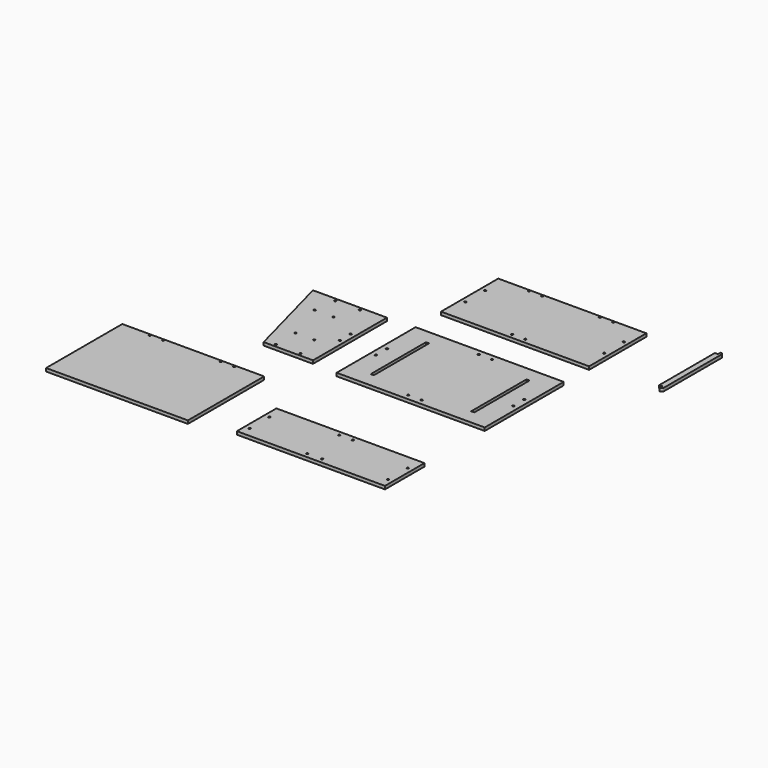
from build123d import *

# Parameters (mm, degrees)
F1_R     = 2
F4_DEPTH = 6.35
F0_R     = 2
F3_R     = 2
F2_R     = 2
F5_DEPTH = 6.35
F6_R     = 2
F7_DEPTH = 6.35


# Not quite as in the source:
# - a feature names something its author has since deleted; it is built from what else it names


with BuildPart() as f4:
    # F1 (on Top) → F4 (new body)
    with BuildSketch(Plane.XY):
        Polygon((1.8228454292, -180.5016371835), (-119.6771545708, -180.5016371835), (-119.6771545708, -210.5016371835), (-119.6771545708, -260.5016371835), (-119.6771545708, -280.5016371835), (30.3228454292, -280.5016371835), (180.3228454292, -280.5016371835), (180.3228454292, -180.5016371835), (58.8228454292, -180.5016371835), (28.8228454292, -180.5016371835), (15.3228454292, -180.5016371835), align=None)
        with Locations((-109.8271545708, -260.5016371835)):
            Circle(F1_R, mode=Mode.SUBTRACT)
        with Locations((15.3228454292, -271.0016371835)):
            Circle(F1_R, mode=Mode.SUBTRACT)
        with Locations((45.0311610582, -270.556012449)):
            Circle(F1_R, mode=Mode.SUBTRACT)
        with Locations((170.4728454292, -260.5016371835)):
            Circle(F1_R, mode=Mode.SUBTRACT)
        with Locations((-109.8271545708, -210.5016371835)):
            Circle(F1_R, mode=Mode.SUBTRACT)
        with Locations((15.3228454292, -190.0016371835)):
            Circle(F1_R, mode=Mode.SUBTRACT)
        with Locations((170.4728454292, -210.5016371835)):
            Circle(F1_R, mode=Mode.SUBTRACT)
        with Locations((42.6017076852, -189.5924542496)):
            Circle(F1_R, mode=Mode.SUBTRACT)
    extrude(amount=F4_DEPTH)


with BuildPart() as f4b:
    # F0 (on Top) → F4, piece 2 (new body)
    with BuildSketch(Plane.XY):
        Polygon((28.5, 174.3550467463), (-121.5, 174.3550467463), (-121.5, 88.3550467463), (-121.5, 60.3550467463), (-121.5, -25.6449532537), (0, -25.6449532537), (57, -25.6449532537), (178.5, -25.6449532537), (178.5, 174.3550467463), align=None)
        with Locations((-110.65, 60.3550467463)):
            Circle(F0_R, mode=Mode.SUBTRACT)
        Polygon((-76.5, 144.3550467463), (-70.15, 144.3550467463), (-70.15, 4.3550467463), (-76.5, 4.3550467463), (-76.5, 44.3550467463), (-76.5, 74.3550467463), align=None, mode=Mode.SUBTRACT)
        with Locations((15, -14.7949532537)):
            Circle(F0_R, mode=Mode.SUBTRACT)
        with Locations((42, -14.7949532537)):
            Circle(F0_R, mode=Mode.SUBTRACT)
        with Locations((-110.65, 88.3550467463)):
            Circle(F0_R, mode=Mode.SUBTRACT)
        with BuildLine():
            ThreePointArc((17, 163.5050467463), (13.5857864376, 162.0908331839), (15, 165.5050467463))
            ThreePointArc((15, 165.5050467463), (16.4142135624, 164.9192603087), (17, 163.5050467463))
        make_face(mode=Mode.SUBTRACT)
        with Locations((42, 163.5050467463)):
            Circle(F0_R, mode=Mode.SUBTRACT)
        Polygon((127.15, 4.3550467463), (127.15, 144.3550467463), (133.5, 144.3550467463), (133.5, 74.3550467463), (133.5, 44.3550467463), (133.5, 4.3550467463), align=None, mode=Mode.SUBTRACT)
        with Locations((167.65, 60.3550467463)):
            Circle(F0_R, mode=Mode.SUBTRACT)
        with Locations((167.65, 88.3550467463)):
            Circle(F0_R, mode=Mode.SUBTRACT)
    extrude(amount=F4_DEPTH)

    # F0 (on Top) → F5 (join)
    with BuildSketch(Plane.XY):
        Polygon((28.5, 174.3550467463), (-121.5, 174.3550467463), (-121.5, 88.3550467463), (-121.5, 60.3550467463), (-121.5, -25.6449532537), (0, -25.6449532537), (57, -25.6449532537), (178.5, -25.6449532537), (178.5, 174.3550467463), align=None)
        with Locations((-110.65, 60.3550467463)):
            Circle(F0_R, mode=Mode.SUBTRACT)
        Polygon((-76.5, 144.3550467463), (-70.15, 144.3550467463), (-70.15, 4.3550467463), (-76.5, 4.3550467463), (-76.5, 44.3550467463), (-76.5, 74.3550467463), align=None, mode=Mode.SUBTRACT)
        with Locations((15, -14.7949532537)):
            Circle(F0_R, mode=Mode.SUBTRACT)
        with Locations((42, -14.7949532537)):
            Circle(F0_R, mode=Mode.SUBTRACT)
        with Locations((-110.65, 88.3550467463)):
            Circle(F0_R, mode=Mode.SUBTRACT)
        with BuildLine():
            ThreePointArc((17, 163.5050467463), (13.5857864376, 162.0908331839), (15, 165.5050467463))
            ThreePointArc((15, 165.5050467463), (16.4142135624, 164.9192603087), (17, 163.5050467463))
        make_face(mode=Mode.SUBTRACT)
        with Locations((42, 163.5050467463)):
            Circle(F0_R, mode=Mode.SUBTRACT)
        Polygon((127.15, 4.3550467463), (127.15, 144.3550467463), (133.5, 144.3550467463), (133.5, 74.3550467463), (133.5, 44.3550467463), (133.5, 4.3550467463), align=None, mode=Mode.SUBTRACT)
        with Locations((167.65, 60.3550467463)):
            Circle(F0_R, mode=Mode.SUBTRACT)
        with Locations((167.65, 88.3550467463)):
            Circle(F0_R, mode=Mode.SUBTRACT)
    extrude(amount=F5_DEPTH)


with BuildPart() as f4c:
    # F3 (on Top) → F4, piece 3 (new body)
    with BuildSketch(Plane.XY):
        Polygon((-46.8814379573, 386.040173464), (-123.3814379573, 386.040173464), (-123.3814379573, 341.040173464), (-123.3814379573, 336.040173464), (-123.3814379573, 291.040173464), (-123.3814379573, 286.040173464), (-123.3814379573, 241.040173464), (-1.8814379573, 241.040173464), (13.1185620427, 241.040173464), (26.6185620427, 241.040173464), (40.1185620427, 241.040173464), (55.1185620427, 241.040173464), (176.6185620427, 241.040173464), (176.6185620427, 386.040173464), (-19.8814379573, 386.040173464), (-31.8814379573, 386.040173464), align=None)
        with Locations((13.1185620427, 250.540173464)):
            Circle(F3_R, mode=Mode.SUBTRACT)
        with Locations((-114.0314379573, 291.040173464)):
            Circle(F3_R, mode=Mode.SUBTRACT)
        with Locations((40.1185620427, 250.540173464)):
            Circle(F3_R, mode=Mode.SUBTRACT)
        with Locations((167.2685620427, 291.040173464)):
            Circle(F3_R, mode=Mode.SUBTRACT)
        with Locations((-114.0314379573, 341.040173464)):
            Circle(F3_R, mode=Mode.SUBTRACT)
        with Locations((-58.8814379573, 383.040173464)):
            Circle(F3_R, mode=Mode.SUBTRACT)
        with BuildLine():
            ThreePointArc((-33.8814379573, 383.040173464), (-33.2956515197, 384.4543870263), (-31.8814379573, 385.040173464))
            ThreePointArc((-31.8814379573, 385.040173464), (-30.4672243949, 384.4543870263), (-29.8814379573, 383.040173464))
            ThreePointArc((-29.8814379573, 383.040173464), (-30.4672243949, 381.6259599016), (-31.8814379573, 381.040173464))
            ThreePointArc((-31.8814379573, 381.040173464), (-33.2956515197, 381.6259599016), (-33.8814379573, 383.040173464))
        make_face(mode=Mode.SUBTRACT)
        with Locations((167.2685620427, 341.040173464)):
            Circle(F3_R, mode=Mode.SUBTRACT)
        with Locations((85.1185620427, 383.040173464)):
            Circle(F3_R, mode=Mode.SUBTRACT)
        with Locations((112.1185620427, 383.040173464)):
            Circle(F3_R, mode=Mode.SUBTRACT)
    extrude(amount=F4_DEPTH)


with BuildPart() as f4d:
    # F2 (on Top) → F4, piece 4 (new body)
    with BuildSketch(Plane.XY):
        Polygon((-282.6041665554, 171.5612447582), (-327.3041665554, 171.5612447582), (-277.3041665554, -15.7387552418), (-257.3041665554, -15.7387552418), (-207.3041665554, -15.7387552418), (-177.3041665554, -15.7387552418), (-177.3041665554, 64.2612447582), (-177.3041665554, 91.5612447582), (-177.3041665554, 171.5612447582), (-208.6041665554, 171.5612447582), (-227.3041665554, 171.5612447582), (-244.6041665554, 171.5612447582), (-246.6041665554, 171.5612447582), (-277.3041665554, 171.5612447582), align=None)
        with Locations((-257.3041665554, -9.7387552418)):
            Circle(F2_R, mode=Mode.SUBTRACT)
        with Locations((-207.3041665554, -9.7387552418)):
            Circle(F2_R, mode=Mode.SUBTRACT)
        with Locations((-257.4761807919, 40.2612447582)):
            Circle(F2_R, mode=Mode.SUBTRACT)
        with Locations((-219.4761807919, 40.2612447582)):
            Circle(F2_R, mode=Mode.SUBTRACT)
        with Locations((-186.8041665554, 64.2612447582)):
            Circle(F2_R, mode=Mode.SUBTRACT)
        with Locations((-186.8041665554, 91.5612447582)):
            Circle(F2_R, mode=Mode.SUBTRACT)
        with Locations((-282.6041665554, 120.2612447582)):
            Circle(F2_R, mode=Mode.SUBTRACT)
        with Locations((-244.6041665554, 120.2612447582)):
            Circle(F2_R, mode=Mode.SUBTRACT)
        with Locations((-277.3041665554, 165.5612447582)):
            Circle(F2_R, mode=Mode.SUBTRACT)
        with Locations((-227.3041665554, 165.5612447582)):
            Circle(F2_R, mode=Mode.SUBTRACT)
    extrude(amount=F4_DEPTH)


with BuildPart() as f5:
    # F0 (on Top) → F5, piece 2 (new body)
    with BuildSketch(Plane.XY):
        with BuildLine():
            Line((309.8231719379, 400.8808784962), (303.4731719379, 400.8808784962))
            Line((303.4731719379, 400.8808784962), (303.4731719379, 260.0808784962))
            Line((303.4731719379, 260.0808784962), (309.8231719379, 260.0808784962))
            Line((309.8231719379, 260.0808784962), (309.8231719379, 253.0808784962))
            ThreePointArc((309.8231719379, 253.0808784962), (313.3587058439, 254.5453445902), (314.8231719379, 258.0808784962))
            Line((314.8231719379, 258.0808784962), (314.8231719379, 402.8808784962))
            ThreePointArc((314.8231719379, 402.8808784962), (313.3587058439, 406.4164124021), (309.8231719379, 407.8808784962))
            Line((309.8231719379, 407.8808784962), (309.8231719379, 400.8808784962))
        make_face()
    extrude(amount=F5_DEPTH)


with BuildPart() as f7:
    # F6 (on Top) → F7 (new body)
    with BuildSketch(Plane.XY):
        Polygon((-405.4018942118, -107.0475112595), (-490.5518942118, -107.0475112595), (-490.5518942118, -300.0475112595), (-203.2518942118, -300.0475112595), (-203.2518942118, -107.0475112595), (-346.9018942118, -107.0475112595), (-378.4018942118, -107.0475112595), align=None)
        with Locations((-432.4018942118, -110.0475112595)):
            Circle(F6_R, mode=Mode.SUBTRACT)
        with Locations((-405.4018942118, -110.0475112595)):
            Circle(F6_R, mode=Mode.SUBTRACT)
        with Locations((-288.4018942118, -110.0475112595)):
            Circle(F6_R, mode=Mode.SUBTRACT)
        with Locations((-261.4018942118, -110.0475112595)):
            Circle(F6_R, mode=Mode.SUBTRACT)
    extrude(amount=F7_DEPTH)


solid = Compound([f4.part, f4b.part, f4c.part, f4d.part, f5.part, f7.part])
